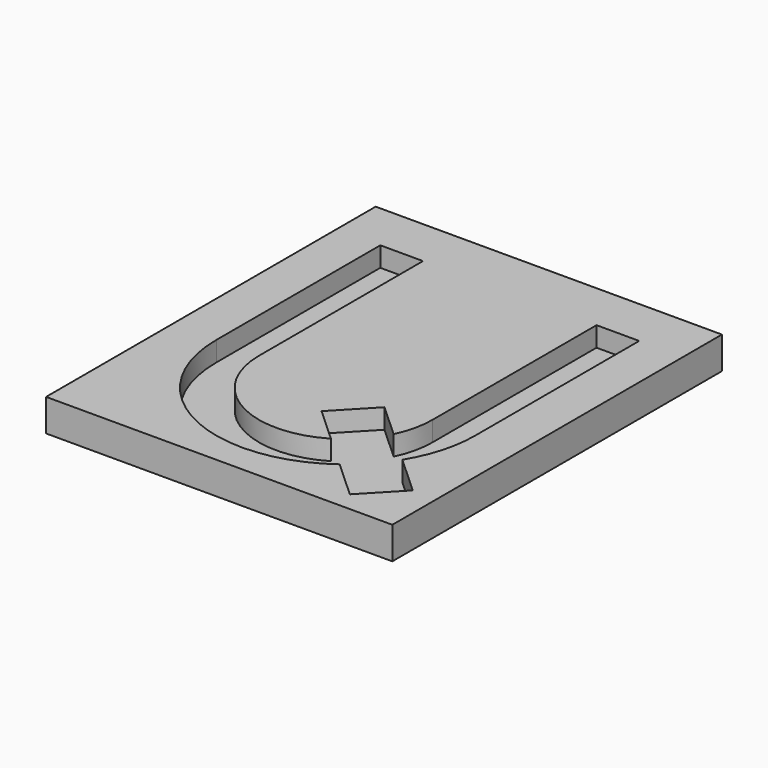
from build123d import *

# Parameters (mm, degrees)
F0_W     = 139.677039
F0_H     = 166.199392
F1_DEPTH = 13
F3_DEPTH = 8


# Not quite as in the source:
# - ends of sketch curves that miss each other by under 0.0002 mm in the source are joined


with BuildPart() as f1:
    # F0 (on Top) → F1 (new body)
    with BuildSketch(Plane.XY):
        with Locations((5e-07, 0)):
            Rectangle(F0_W, F0_H)
    extrude(amount=F1_DEPTH)

    # F2 (on face) → F3 (cut)
    with BuildSketch(Plane.XY.offset(13)):
        with BuildLine():
            Line((-52.224, 63.413361), (-52.224, -19.296639))
            ThreePointArc((-52.224, -19.296639), (-23.4870244983, -65.9411012245), (31.0980686358, -61.2520475086))
            Line((31.0980686358, -61.2520475086), (46.412829, -75.243303))
            Line((46.412829, -75.243303), (60.220039, -60.767602))
            Line((60.220039, -60.767602), (44.587774, -46.486281))
            ThreePointArc((44.587774, -46.486281), (50.2787135157, -33.4174443314), (52.224, -19.296639))
            Line((52.224, -19.296639), (52.224, 63.413361))
            Line((52.224, 63.413361), (35, 63.413361))
            Line((35, 63.413361), (35, -19.296639))
            ThreePointArc((35, -19.296639), (34.1157796878, -27.1141562719), (31.5077956402, -34.536678826))
            Line((31.5077956402, -34.536678826), (17.818477, -22.030395))
            Line((17.818477, -22.030395), (4.000974, -36.496692))
            Line((4.000974, -36.496692), (18.018091, -49.302445))
            ThreePointArc((18.018091, -49.302445), (-17.2390082984, -49.756720958), (-35, -19.296639))
            Line((-35, -19.296639), (-35, 63.413361))
            Line((-35, 63.413361), (-52.224, 63.413361))
        make_face()
    extrude(amount=-F3_DEPTH, mode=Mode.SUBTRACT)


solid = f1.part
